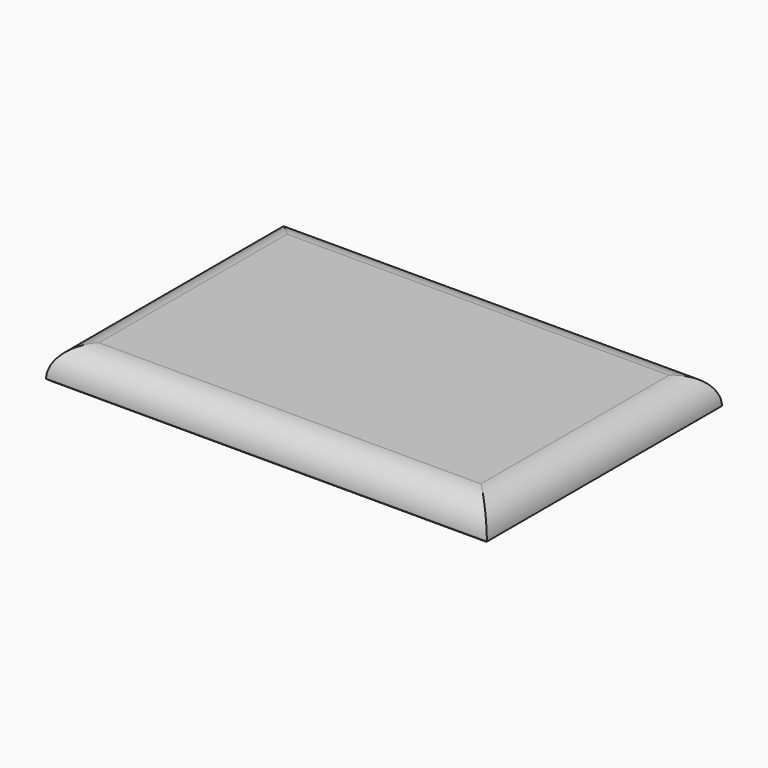
from build123d import *

# Parameters (mm, degrees)
F0_W        = 76.2
F0_H        = 50.8
F1_DEPTH    = 6.35
F2_R        = 5.08
F3_T1_DEPTH = 93.0005208253
F3_T3_DEPTH = 67.6005208253


# Not quite as in the source:
# - a fillet or chamfer that OpenCascade refuses, or shapes differently, is made with other operations: its cross-section is extruded or revolved along the edge and cut away or added


with BuildPart() as f1:
    # F0 (on Top) → F1 (new body)
    with BuildSketch(Plane.XY):
        with Locations((38.1, -25.4)):
            Rectangle(F0_W, F0_H)
    extrude(amount=F1_DEPTH)

    # F2
    f2_edges = [f1.edges().sort_by_distance(p)[0] for p in [
        (38.1, 0, 6.35),
        (0, -25.4, 6.35),
        (38.1, -50.8, 6.35),
        (76.2, -25.4, 6.35),
    ]]
    fillet(f2_edges, radius=F2_R)

    # F3: fillet of radius 5.08 on 4 edges, made by hand

    # F3_s2 → F3_t1 (cut)
    with BuildSketch(Plane.YZ.offset(-8.4002604126)):
        with BuildLine():
            add(Edge.make_bspline(
                [(0, 1.27), (-1.4400446422, 0), (-3.3601041651, 0)],
                knots=[0, 0, 0, 1, 1, 1], degree=2, weights=[1, 1, 1]))
            Line((-3.3601041651, 0), (0, 0))
            Line((0, 0), (0, 1.27))
        make_face()
        with BuildLine():
            add(Edge.make_bspline(
                [(-47.4398958349, 0), (-49.3599553578, 0), (-50.8, 1.27)],
                knots=[0, 0, 0, 1, 1, 1], degree=2, weights=[1, 1, 1]))
            Line((-50.8, 1.27), (-50.8, 0))
            Line((-50.8, 0), (-47.4398958349, 0))
        make_face()
    extrude(amount=F3_T1_DEPTH, mode=Mode.SUBTRACT)

    # F3_s4 → F3_t3 (cut)
    with BuildSketch(Plane.XZ.offset(-8.4002604126)):
        with BuildLine():
            add(Edge.make_bspline(
                [(3.3601041651, 0), (1.4400446422, 0), (0, 1.27)],
                knots=[0, 0, 0, 1, 1, 1], degree=2, weights=[1, 1, 1]))
            Line((0, 1.27), (0, 0))
            Line((0, 0), (3.3601041651, 0))
        make_face()
        with BuildLine():
            add(Edge.make_bspline(
                [(76.2, 1.27), (74.7599553578, 0), (72.8398958349, 0)],
                knots=[0, 0, 0, 1, 1, 1], degree=2, weights=[1, 1, 1]))
            Line((72.8398958349, 0), (76.2, 0))
            Line((76.2, 0), (76.2, 1.27))
        make_face()
    extrude(amount=F3_T3_DEPTH, mode=Mode.SUBTRACT)


solid = f1.part
